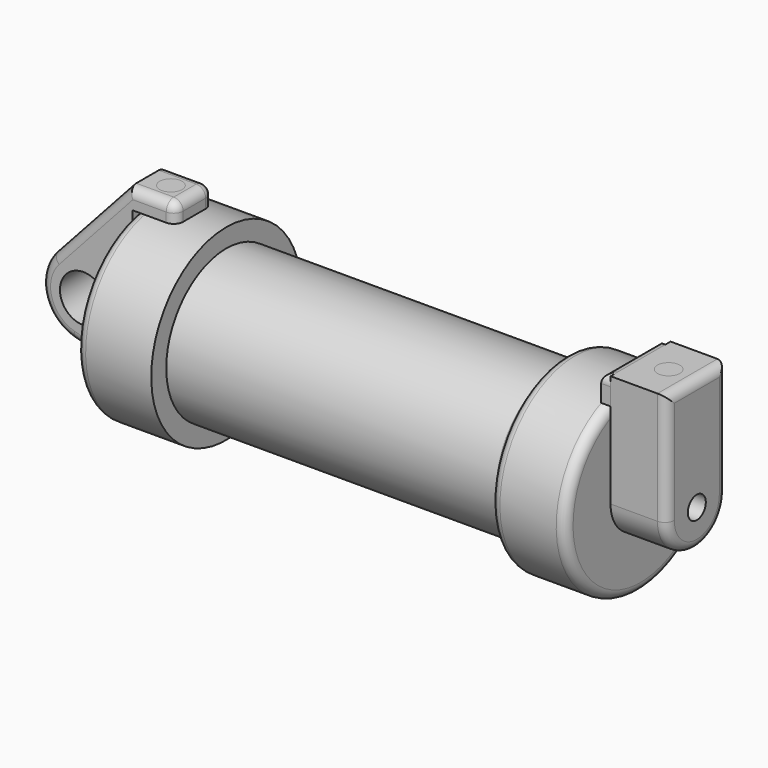
from build123d import *

# Parameters (mm, degrees)
F0_W     = 5.842
F0_H     = 12.7
F0_R     = 3.175
F2_DEPTH = 3.175
F3_R     = 1.524
F4_DEPTH = 7.62
F5_DEPTH = 1.27
F6_R     = 1.524
F7_DEPTH = 10.414
F8_R     = 1.524
F9_DEPTH = 17.78
F10_R    = 1.26999
F10_2_R  = 1.26999
F10_3_R  = 1.26999
F10_4_R  = 1.26999


# Not quite as in the source:
# - a fillet or chamfer is up to 0.001 mm smaller than in the source, because OpenCascade refuses the exact size


with BuildPart() as f1:
    # F0 (on Front) → F1 (revolve)
    with BuildSketch(Plane.XZ):
        Polygon((5.842, 12.7), (5.842, 0), (66.294, 0), (66.294, 12.7), (56.134, 12.7), (56.134, 10.16), (10.16, 10.16), (10.16, 12.7), align=None)
        with Locations((2.921, 6.35)):
            Rectangle(F0_W, F0_H)
    revolve(axis=Axis((33.147, 0, 0), (-1, 0, 0)))

    # F10 (radius 1.27 in the source; OpenCascade refuses exactly that, so slightly less here)
    f10_edges = [f1.edges().sort_by_distance(p)[0] for p in [
        (66.294, 0, -12.7),
        (0, 0, -12.7),
        (56.134, 0, -12.7),
        (56.134, 0, -10.16),
    ]]
    fillet(f10_edges, radius=F10_R)


with BuildPart() as f2:
    # F0 (on Front) → F2 (new body, symmetric)
    with BuildSketch(Plane.XZ):
        with BuildLine():
            Line((-0.9398, 0), (0, 0))
            Line((0, 0), (0, 12.7))
            Line((0, 12.7), (5.842, 12.7))
            Line((5.842, 12.7), (5.842, 15.24))
            Line((5.842, 15.24), (-0.508, 15.24))
            Line((-0.508, 15.24), (-10.8806298187, 3.8475430269))
            ThreePointArc((-10.8806298187, 3.8475430269), (-4.5919612295, 5.3297205562), (-0.9398, 0))
        make_face()
        with BuildLine():
            Line((5.842, 0), (0, 0))
            Line((0, 0), (-0.9398, 0))
            ThreePointArc((-0.9398, 0), (-3.1957909266, -4.5493385486), (-8.1826630726, -5.5069827884))
            Line((-8.1826630726, -5.5069827884), (5.842, -9.398))
            Line((5.842, -9.398), (5.842, 0))
        make_face()
        with BuildLine():
            ThreePointArc((-8.1826630726, -5.5069827884), (-3.1957909266, -4.5493385486), (-0.9398, 0))
            ThreePointArc((-0.9398, 0), (-4.5919612295, 5.3297205562), (-10.8806298187, 3.8475430269))
            ThreePointArc((-10.8806298187, 3.8475430269), (-12.1459778134, -1.5837270034), (-8.1826630726, -5.5069827884))
        make_face()
        with Locations((-6.6548, 0)):
            Circle(F0_R, mode=Mode.SUBTRACT)
    extrude(amount=F2_DEPTH, both=True)

    # F10#2 (radius 1.27 in the source; OpenCascade refuses exactly that, so slightly less here)
    f10_2_edges = [f2.edges().sort_by_distance(p)[0] for p in [
        (-12.145978, 3.175, -1.583727),
        (-5.694315, 3.175, 9.543772),
        (-5.694315, -3.175, 9.543772),
        (-12.145978, -3.175, -1.583727),
        (2.667, 3.175, 15.24),
        (2.667, -3.175, 15.24),
        (5.842, 0, 15.24),
        (5.842, -3.175, 13.97),
        (5.842, -3.175, -4.699),
        (5.842, 3.175, 13.97),
        (5.842, 3.175, -4.699),
        (-1.170332, 3.175, -7.452491),
        (-1.170332, -3.175, -7.452491),
    ]]
    fillet(f10_2_edges, radius=F10_2_R)


with BuildPart() as f4:
    # F3 (on face) → F4 (new body)
    with BuildSketch(Plane.YZ.offset(66.294)):
        with BuildLine():
            ThreePointArc((-5.08, 0), (0, -5.08), (5.08, 0))
            ThreePointArc((5.08, 0), (0, 5.08), (-5.08, 0))
        make_face()
        Circle(F3_R, mode=Mode.SUBTRACT)
        with BuildLine():
            ThreePointArc((-5.08, 0), (0, 5.08), (5.08, 0))
            Line((5.08, 0), (5.08, 15.24))
            Line((5.08, 15.24), (-5.08, 15.24))
            Line((-5.08, 15.24), (-5.08, 0))
        make_face()
    extrude(amount=F4_DEPTH)

    # F10#3 (radius 1.27 in the source; OpenCascade refuses exactly that, so slightly less here)
    f10_3_edges = [f4.edges().sort_by_distance(p)[0] for p in [
        (73.914, 5.08, 7.62),
        (73.914, 0, 15.24),
        (73.914, 0, -5.08),
        (73.914, -5.08, 7.62),
    ]]
    fillet(f10_3_edges, radius=F10_3_R)


with BuildPart() as f5:
    # F3 (on face) → F5 (new body)
    with BuildSketch(Plane.YZ.offset(66.294)):
        with BuildLine():
            ThreePointArc((-5.08, 11.6397422652), (0, 12.7), (5.08, 11.6397422652))
            Line((5.08, 11.6397422652), (5.08, 15.24))
            Line((5.08, 15.24), (-5.08, 15.24))
            Line((-5.08, 15.24), (-5.08, 11.6397422652))
        make_face()
    extrude(amount=-F5_DEPTH)

    # F10#4 (radius 1.27 in the source; OpenCascade refuses exactly that, so slightly less here)
    f10_4_edges = [f5.edges().sort_by_distance(p)[0] for p in [
        (65.024, 0, 15.24),
        (65.659, -5.08, 15.24),
        (65.659, 5.08, 15.24),
    ]]
    fillet(f10_4_edges, radius=F10_4_R)


with BuildPart() as f7:
    # F6 (on face) → F7 (new body)
    with BuildSketch(Plane.XY.offset(15.24)):
        with Locations((70.104, 0)):
            Circle(F6_R)
    extrude(amount=-F7_DEPTH)


with BuildPart() as f9:
    # F8 (on face) → F9 (new body)
    with BuildSketch(Plane.XY.offset(15.24)):
        with Locations((2.667, 0)):
            Circle(F8_R)
    extrude(amount=-F9_DEPTH)


solid = Compound([f1.part, f2.part, f4.part, f5.part, f7.part, f9.part])
